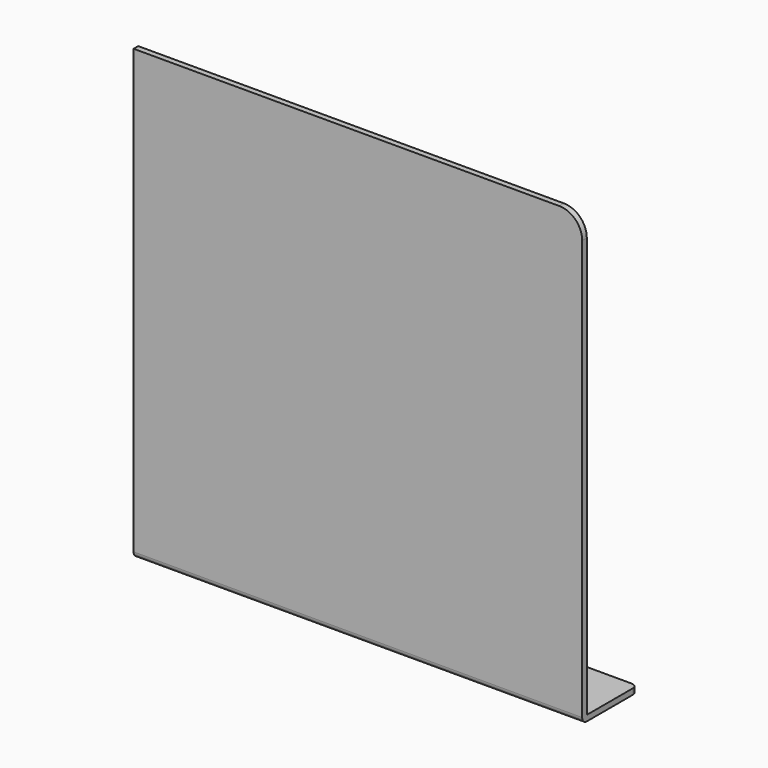
from build123d import *

# Parameters (mm, degrees)
F1_DEPTH = 78
F2_R     = 4
F3_R     = 1


# Not quite as in the source:
# - two fillets or chamfers of one size are made in one step


with BuildPart() as f1:
    # F0 (on Right) → F1 (new body)
    with BuildSketch(Plane.YZ):
        Polygon((0, 78), (0, 0), (12, 0), (12, 1), (1, 1), (1, 78), align=None)
    extrude(amount=F1_DEPTH)

    # F2
    f2_edges = [f1.edges().sort_by_distance(p)[0] for p in [
        (78, 0.5, 78),
    ]]
    fillet(f2_edges, radius=F2_R)

    # F3
    f3_edges = [f1.edges().sort_by_distance(p)[0] for p in [
        (0, 12, 0.5),
        (39, 0, 0),
        (78, 12, 0.5),
    ]]
    fillet(f3_edges, radius=F3_R)


solid = f1.part
